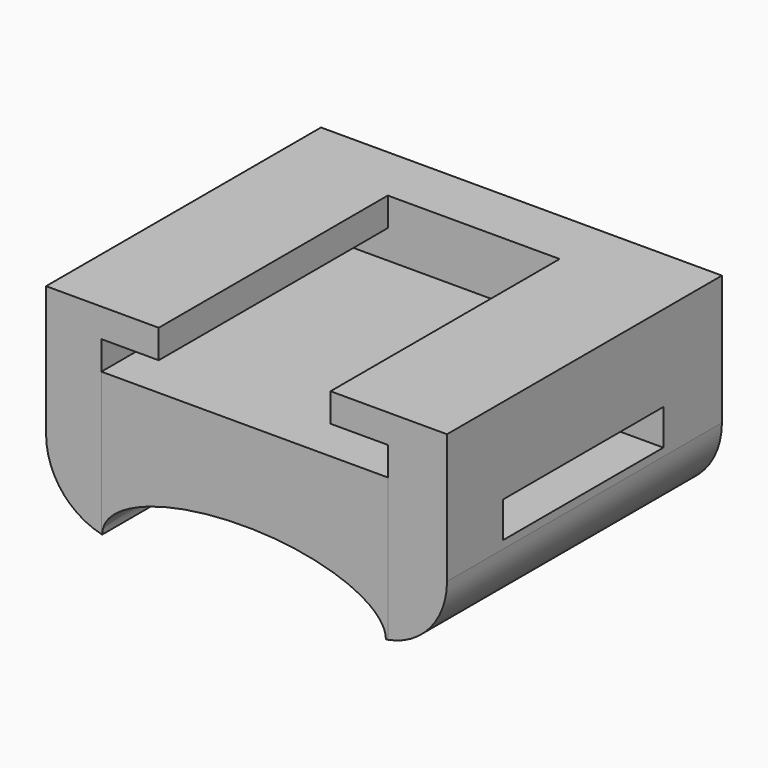
from build123d import *

# Parameters (mm, degrees)
F0_W          = 4
F0_H          = 19.9986558093
F0_W_2        = 12
F0_H_2        = 0.0013441907
F1_DEPTH      = 10
F2_DEPTH      = 14
F3_START      = 12
F3_DEPTH      = 2
F4_W          = 14
F4_H          = 2.5
F5_DEPTH      = 25
F5_DEPTH_BACK = 25
F7_DEPTH      = 25
F7_DEPTH_BACK = 25
F8_T1_DEPTH   = 22.5250523131
F8_T3_DEPTH   = 26.207315151
F8_T5_DEPTH   = 26.047082038
F8_T7_DEPTH   = 22.364820273


# Not quite as in the source:
# - a fillet or chamfer that OpenCascade refuses, or shapes differently, is made with other operations: its cross-section is extruded or revolved along the edge and cut away or added


with BuildPart() as f1:
    # F0 (on Top) → F1 (new body)
    with BuildSketch(Plane.XY):
        Polygon((-9.9598446302, -10.1588685066), (-9.9598446302, 9.8397873028), (-5.9598446302, 9.8397873028), (6.0401553698, 9.8397873028), (10.0401553698, 9.8397873028), (10.0401553698, -10.1588685066), (14.174235519, -10.1588685066), (14.174235519, 13.8411314934), (-13.825764481, 13.8411314934), (-13.825764481, -10.1588685066), align=None)
        with Locations((-7.9598446302, -0.1595406019)):
            Rectangle(F0_W, F0_H)
        with Locations((0.0401553698, -0.1595406019)):
            Rectangle(F0_W_2, F0_H)
        with Locations((-7.9598446302, -10.1595406019)):
            Rectangle(F0_W, F0_H_2)
        with Locations((8.0401553698, -0.1595406019)):
            Rectangle(F0_W, F0_H)
        with Locations((0.0401553698, -10.1595406019)):
            Rectangle(F0_W_2, F0_H_2)
        with Locations((8.0401553698, -10.1595406019)):
            Rectangle(F0_W, F0_H_2)
    extrude(amount=F1_DEPTH)

    # F0 (on Top) → F2 (join)
    with BuildSketch(Plane.XY):
        Polygon((-9.9598446302, -10.1588685066), (-9.9598446302, 9.8397873028), (-5.9598446302, 9.8397873028), (6.0401553698, 9.8397873028), (10.0401553698, 9.8397873028), (10.0401553698, -10.1588685066), (14.174235519, -10.1588685066), (14.174235519, 13.8411314934), (-13.825764481, 13.8411314934), (-13.825764481, -10.1588685066), align=None)
    extrude(amount=F2_DEPTH)

    # F0 (on Top) → F3 (join)
    with BuildSketch(Plane.XY.offset(F3_START)):
        with Locations((8.0401553698, -0.1595406019)):
            Rectangle(F0_W, F0_H)
        with Locations((-7.9598446302, -0.1595406019)):
            Rectangle(F0_W, F0_H)
    extrude(amount=F3_DEPTH)

    # F4 (on Right) → F5 (cut, two sides)
    with BuildSketch(Plane.YZ) as f5_sk:
        with Locations((1.7279156186, 6.75)):
            Rectangle(F4_W, F4_H)
    extrude(amount=-F5_DEPTH, mode=Mode.SUBTRACT)
    extrude(f5_sk.sketch, amount=F5_DEPTH_BACK, mode=Mode.SUBTRACT)

    # F6 (on Front) → F7 (cut, two sides)
    with BuildSketch(Plane.XZ) as f7_sk:
        with BuildLine():
            add(Edge.make_bspline(
                [(9.9038929624, 0), (9.9038929624, 6.5060013768), (-4.9519464812, 3.2530006884), (-19.8077859248, 0), (-4.9519464812, -3.2530006884), (9.9038929624, -6.5060013768), (9.9038929624, 0)],
                knots=[0, 0, 0, 2.0943951024, 2.0943951024, 4.1887902048, 4.1887902048, 6.2831853072, 6.2831853072, 6.2831853072], degree=2, weights=[1, 0.5, 1, 0.5, 1, 0.5, 1]))
        make_face()
    extrude(amount=-F7_DEPTH, mode=Mode.SUBTRACT)
    extrude(f7_sk.sketch, amount=F7_DEPTH_BACK, mode=Mode.SUBTRACT)

    # F8: fillet of radius 5 on 2 edges, made by hand

    # F8_s2 → F8_t1 (cut)
    with BuildSketch(Plane.XZ.offset(-7.45e-08)):
        with BuildLine():
            ThreePointArc((14.174235519, 4.9464734928), (12.9589605564, 1.6790805885), (9.9038929624, 0))
            Line((9.9038929624, 0), (14.174235519, 0))
            Line((14.174235519, 0), (14.174235519, 4.9464734928))
        make_face()
    extrude(amount=F8_T1_DEPTH, mode=Mode.SUBTRACT)

    # F8_s4 → F8_t3 (cut)
    with BuildSketch(Plane.XZ.offset(-26.2073152255)):
        with BuildLine():
            ThreePointArc((14.174235519, 4.9464734928), (12.9589605564, 1.6790805885), (9.9038929624, 0))
            Line((9.9038929624, 0), (14.174235519, 0))
            Line((14.174235519, 0), (14.174235519, 4.9464734928))
        make_face()
    extrude(amount=F8_T3_DEPTH, mode=Mode.SUBTRACT)

    # F8_s6 → F8_t5 (cut)
    with BuildSketch(Plane.XZ.offset(-26.0470826489)):
        with BuildLine():
            ThreePointArc((-13.825764481, 4.8823804622), (-12.7238821297, 1.7511380895), (-9.9038929624, 0))
            Line((-9.9038929624, 0), (-13.825764481, 0))
            Line((-13.825764481, 0), (-13.825764481, 4.8823804622))
        make_face()
    extrude(amount=F8_T5_DEPTH, mode=Mode.SUBTRACT)

    # F8_s8 → F8_t7 (cut)
    with BuildSketch(Plane.XZ.offset(-6.109e-07)):
        with BuildLine():
            ThreePointArc((-13.825764481, 4.8823804622), (-12.7238821297, 1.7511380895), (-9.9038929624, 0))
            Line((-9.9038929624, 0), (-13.825764481, 0))
            Line((-13.825764481, 0), (-13.825764481, 4.8823804622))
        make_face()
    extrude(amount=F8_T7_DEPTH, mode=Mode.SUBTRACT)


solid = f1.part
